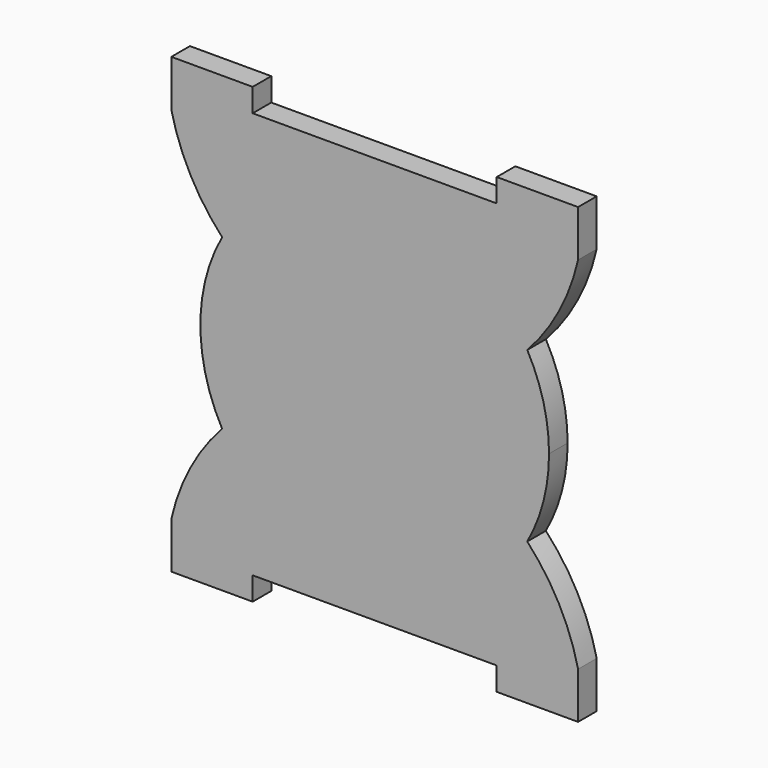
from build123d import *

# Parameters (mm, degrees)
F1_DEPTH = 2


with BuildPart() as f1:
    # F0 (on Front) → F1 (new body)
    with BuildSketch(Plane.XZ):
        with BuildLine():
            ThreePointArc((13.1280048062, -7.2564102564), (14.5244633652, -3.746993989), (15, 0))
            ThreePointArc((15, 0), (14.5244633652, 3.746993989), (13.1280048062, 7.2564102564))
            ThreePointArc((13.1280048062, 7.2564102564), (0, 1.548676929), (-13.1280048062, 7.2564102564))
            ThreePointArc((-13.1280048062, 7.2564102564), (-15, 0), (-13.1280048062, -7.2564102564))
            ThreePointArc((-13.1280048062, -7.2564102564), (0, -1.548676929), (13.1280048062, -7.2564102564))
        make_face()
        with BuildLine():
            ThreePointArc((-13.1280048062, 7.2564102564), (0, 1.548676929), (13.1280048062, 7.2564102564))
            ThreePointArc((13.1280048062, 7.2564102564), (0, 15), (-13.1280048062, 7.2564102564))
        make_face()
        with BuildLine():
            ThreePointArc((-13.1280048062, 7.2564102564), (0, 15), (13.1280048062, 7.2564102564))
            ThreePointArc((13.1280048062, 7.2564102564), (15.8589994188, 11.0891654734), (17.5, 15.5))
            Line((17.5, 15.5), (17.5, 19.5))
            Line((17.5, 19.5), (10.5, 19.5))
            Line((10.5, 19.5), (10.5, 17.5))
            Line((10.5, 17.5), (-10.5, 17.5))
            Line((-10.5, 17.5), (-10.5, 19.5))
            Line((-10.5, 19.5), (-17.5, 19.5))
            Line((-17.5, 19.5), (-17.5, 15.5))
            ThreePointArc((-17.5, 15.5), (-15.8589994188, 11.0891654734), (-13.1280048062, 7.2564102564))
        make_face()
        with BuildLine():
            ThreePointArc((17.5, -15.5), (15.8589994188, -11.0891654734), (13.1280048062, -7.2564102564))
            ThreePointArc((13.1280048062, -7.2564102564), (0, -15), (-13.1280048062, -7.2564102564))
            ThreePointArc((-13.1280048062, -7.2564102564), (-15.8589994188, -11.0891654734), (-17.5, -15.5))
            Line((-17.5, -15.5), (-17.5, -19.5))
            Line((-17.5, -19.5), (-10.5, -19.5))
            Line((-10.5, -19.5), (-10.5, -17.5))
            Line((-10.5, -17.5), (10.5, -17.5))
            Line((10.5, -17.5), (10.5, -19.5))
            Line((10.5, -19.5), (17.5, -19.5))
            Line((17.5, -19.5), (17.5, -15.5))
        make_face()
        with BuildLine():
            ThreePointArc((-13.1280048062, -7.2564102564), (0, -15), (13.1280048062, -7.2564102564))
            ThreePointArc((13.1280048062, -7.2564102564), (0, -1.548676929), (-13.1280048062, -7.2564102564))
        make_face()
    extrude(amount=F1_DEPTH)


solid = f1.part
